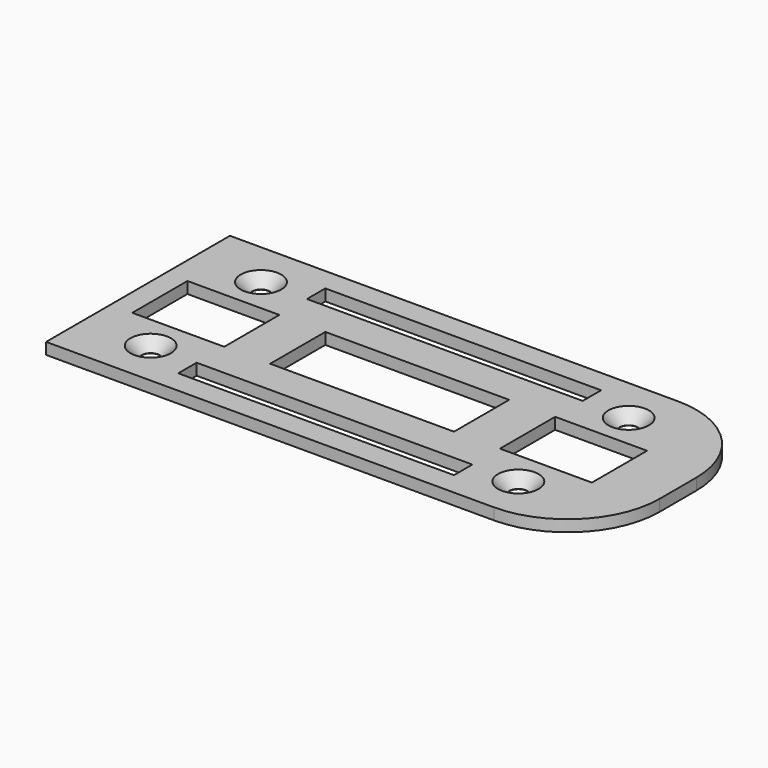
from build123d import *
from build123d import SkipClean  # not in build123d's __all__

# Parameters (mm, degrees)
F1_DEPTH        = 31.75
F1_DEPTH_BACK   = 31.75
F3_R            = 6.35
F4_DEPTH        = 149.1828857926
F5_R            = 12.7
F6_DEPTH        = 25.4
F7_R            = 9.525
F8_DEPTH        = 44.45
F8_DEPTH_BACK   = 66.9427915833
F10_D           = 4.2
F10_DEPTH       = 25.4
F10_TIP         = 1.2618073
F12_DEPTH       = 3.175
F14_D           = 5
F14_CSINK_D     = 11.2
F14_CSINK_ANGLE = 90
F15_W           = 25.4
F15_H           = 19.05
F15_W_2         = 76.2
F15_H_2         = 6.35
F15_W_3         = 50.8
F16_DEPTH       = 41.2760001


# Not quite as in the source:
# - a feature of the source that left no trace in its solid (it failed there, or was rolled back) is left out


with BuildPart() as f1:
    # F0 (on Front) → F1 (new body, two sides)
    with BuildSketch(Plane.XZ) as f1_sk:
        with BuildLine():
            Line((66.9417914833, 19.05), (-82.2400942093, 19.05))
            Line((-82.2400942093, 19.05), (-82.2400942093, -19.05))
            add(Edge.make_bspline(
                [(-82.2400942093, -19.05), (0, -19.05), (66.9417914833, -19.05), (66.9417914833, 19.05)],
                knots=[0, 0, 0, 0, 153.970273166, 153.970273166, 153.970273166, 153.970273166], degree=3))
        make_face()
    extrude(amount=F1_DEPTH)
    extrude(f1_sk.sketch, amount=-F1_DEPTH_BACK)

    # F3 (on face) → F4 (cut, through all)
    with BuildSketch(Plane(origin=(-82.2400942093, 0, 0), x_dir=(0, -1, 0), z_dir=(-1, 0, 0))):
        Circle(F3_R)
    extrude(amount=-F4_DEPTH, mode=Mode.SUBTRACT)

    # F5 (on face) → F6 (cut)
    with BuildSketch(Plane(origin=(-82.2400942093, 0, 0), x_dir=(0, -1, 0), z_dir=(-1, 0, 0))):
        Circle(F5_R)
    extrude(amount=-F6_DEPTH, mode=Mode.SUBTRACT)

    # F7 (on Right) → F8 (cut, two sides)
    with BuildSketch(Plane.YZ) as f8_sk:
        Circle(F7_R)
    extrude(amount=-F8_DEPTH, mode=Mode.SUBTRACT)
    extrude(f8_sk.sketch, amount=F8_DEPTH_BACK, mode=Mode.SUBTRACT)

    # F10
    with Locations(Plane.XY.offset(19.05)):
        with Locations((-63.5, 19.05), (-63.5, -19.05), (25.4, 19.05), (25.4, -19.05)):
            Hole(F10_D / 2, depth=F10_DEPTH)
            with Locations((0, 0, -(F10_DEPTH + F10_TIP / 2))):  # 118° drill point
                Cone(0, F10_D / 2, F10_TIP, mode=Mode.SUBTRACT)


with BuildPart() as f12:
    # F11 (on face) → F12 (new body)
    with BuildSketch(Plane.XY.offset(19.05)):
        with BuildLine():
            Line((41.5417914833, 31.75), (-82.2400942093, 31.75))
            Line((-82.2400942093, 31.75), (-82.2400942093, -31.75))
            Line((-82.2400942093, -31.75), (41.5417914833, -31.75))
            ThreePointArc((41.5417914833, -31.75), (59.5023037254, -24.3105122421), (66.9417914833, -6.35))
            Line((66.9417914833, -6.35), (66.9417914833, 6.35))
            ThreePointArc((66.9417914833, 6.35), (59.5023037254, 24.3105122421), (41.5417914833, 31.75))
        make_face()
    extrude(amount=F12_DEPTH)

    # F14 (through all)
    with Locations(Plane.XY.offset(22.225)):
        with Locations((-63.5, 19.05), (-63.5, -19.05), (38.1, -19.05), (38.1, 19.05)):
            CounterSinkHole(F14_D / 2, F14_CSINK_D / 2, counter_sink_angle=F14_CSINK_ANGLE)


with BuildPart() as f16_tool:
    # F15 (on face) → F16 (new body, through all)
    with BuildSketch(Plane.XY.offset(22.225)):
        with Locations((-63.5, 0)):
            Rectangle(F15_W, F15_H)
        with Locations((38.1, 0)):
            Rectangle(F15_W, F15_H)
        with Locations((-12.7, 22.225)):
            Rectangle(F15_W_2, F15_H_2)
        with Locations((-12.7, -22.225)):
            Rectangle(F15_W_2, F15_H_2)
        with Locations((-12.7, 0)):
            Rectangle(F15_W_3, F15_H)
    extrude(amount=-F16_DEPTH)


with BuildPart() as f1_1:
    add(f1.part, clean=False)

    # F16: cut by f16_tool
    with SkipClean():  # cleaning this boolean's faces spoils the solid; the shape is the same uncleaned
        add(f16_tool.part, mode=Mode.SUBTRACT)


with BuildPart() as f12_1:
    add(f12.part, clean=False)

    # F16: cut by f16_tool
    with SkipClean():  # cleaning this boolean's faces spoils the solid; the shape is the same uncleaned
        add(f16_tool.part, mode=Mode.SUBTRACT)


solid = f12_1.part
